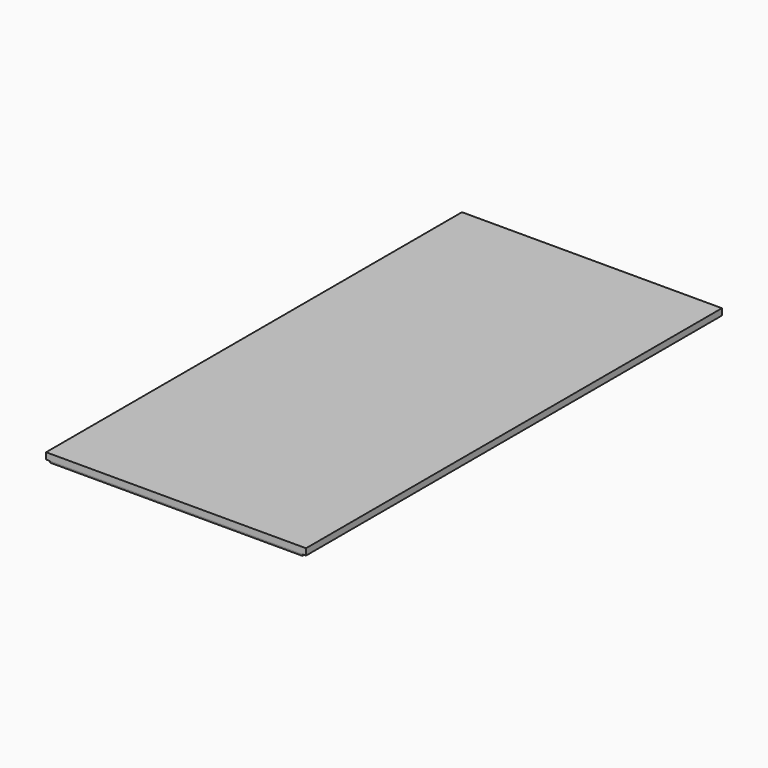
from build123d import *

# Parameters (mm, degrees)
F0_W     = 863.6
F0_H     = 1778
F1_DEPTH = 4.7625
F2_DEPTH = 4.7625
F3_W     = 889
F3_H     = 1778
F4_DEPTH = 22.225


# Not quite as in the source:
# - a length typed as a fraction of an inch, garbled in the dataset ("3 / 203.2 mm" for 3/8 in), is restored


with BuildPart() as f1:
    # F0 (on Top) → F1 (new body)
    with BuildSketch(Plane.XY):
        with Locations((-85.0043228032, 2.0000711083)):
            Rectangle(F0_W, F0_H)
    extrude(amount=F1_DEPTH)

    # F2 (add): a face of the model
    f2_faces = [f1.faces().sort_by_distance(p)[0] for p in [
        (-85.0043228032, 2.0000711083, 4.7625),
    ]]
    extrude(f2_faces, amount=-F2_DEPTH)


with BuildPart() as f4:
    # F3 (on Top) → F4 (new body)
    with BuildSketch(Plane.XY):
        with Locations((-97.7043228032, 2.0000711083)):
            Rectangle(F3_W, F3_H)
    extrude(amount=F4_DEPTH)


with BuildPart() as f1_1:
    # F5: moved
    add(f1.part.moved(Location((-12.7, 0, -4.7625))))


solid = Compound([f4.part, f1_1.part])
